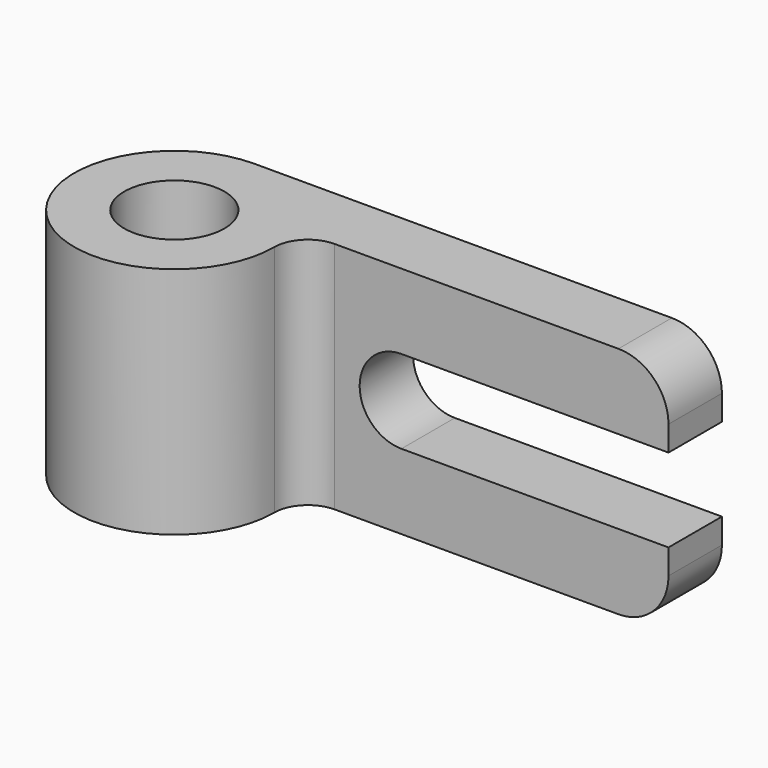
from build123d import *

# Parameters (mm, degrees)
F0_R     = 9.525
F1_DEPTH = 44.45
F2_R     = 6.34999
F4_DEPTH = 12.7
F5_R     = 9.525


# Not quite as in the source:
# - a fillet or chamfer is up to 0.001 mm smaller than in the source, because OpenCascade refuses the exact size


with BuildPart() as f1:
    # F0 (on Top) → F1 (new body)
    with BuildSketch(Plane.XY):
        with BuildLine():
            ThreePointArc((0, 19.05), (-13.4703841816, -13.4703841816), (19.05, 0))
            Line((19.05, 0), (19.05, 6.35))
            Line((19.05, 6.35), (17.9605122421, 6.35))
            ThreePointArc((17.9605122421, 6.35), (10.9985226281, 15.5542598667), (0, 19.05))
        make_face()
        Circle(F0_R, mode=Mode.SUBTRACT)
        with BuildLine():
            Line((38.1, 19.05), (0, 19.05))
            ThreePointArc((0, 19.05), (10.9985226281, 15.5542598667), (17.9605122421, 6.35))
            Line((17.9605122421, 6.35), (19.05, 6.35))
            Line((19.05, 6.35), (38.1, 6.35))
            Line((38.1, 6.35), (88.9, 6.35))
            Line((88.9, 6.35), (88.9, 19.05))
            Line((88.9, 19.05), (38.1, 19.05))
        make_face()
    extrude(amount=F1_DEPTH)

    # F2 (radius 6.35 in the source; OpenCascade refuses exactly that, so slightly less here)
    f2_edges = [f1.edges().sort_by_distance(p)[0] for p in [
        (19.05, 6.35, 22.225),
    ]]
    fillet(f2_edges, radius=F2_R)

    # F3 (on face) → F4 (cut)
    with BuildSketch(Plane.XZ.offset(-6.35)):
        with BuildLine():
            Line((88.9, 14.2875), (88.9, 30.1625))
            Line((88.9, 30.1625), (38.1, 30.1625))
            ThreePointArc((38.1, 30.1625), (43.7126600757, 27.8376600757), (46.0375, 22.225))
            ThreePointArc((46.0375, 22.225), (43.7126600757, 16.6123399243), (38.1, 14.2875))
            Line((38.1, 14.2875), (88.9, 14.2875))
        make_face()
        with BuildLine():
            ThreePointArc((46.0375, 22.225), (43.7126600757, 27.8376600757), (38.1, 30.1625))
            Line((38.1, 30.1625), (38.1, 22.225))
            Line((38.1, 22.225), (38.1, 14.2875))
            ThreePointArc((38.1, 14.2875), (43.7126600757, 16.6123399243), (46.0375, 22.225))
        make_face()
        with BuildLine():
            Line((38.1, 22.225), (38.1, 30.1625))
            ThreePointArc((38.1, 30.1625), (30.1625, 22.225), (38.1, 14.2875))
            Line((38.1, 14.2875), (38.1, 22.225))
        make_face()
    extrude(amount=-F4_DEPTH, mode=Mode.SUBTRACT)

    # F5
    f5_edges = [f1.edges().sort_by_distance(p)[0] for p in [
        (88.9, 12.7, 44.45),
        (88.9, 12.7, 0),
    ]]
    fillet(f5_edges, radius=F5_R)


solid = f1.part
